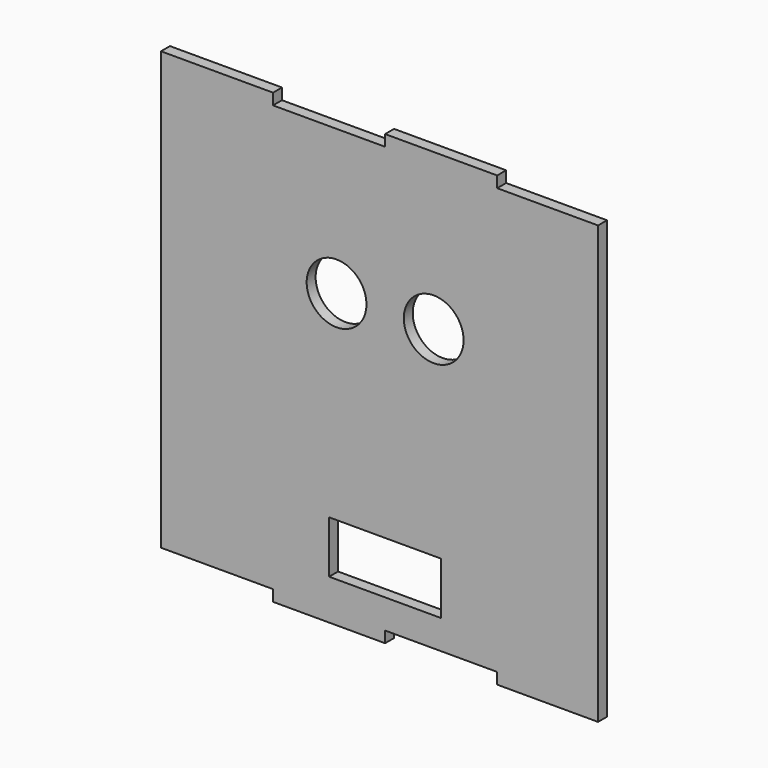
from build123d import *

# Parameters (mm, degrees)
F0_W     = 30
F0_H     = 14
F0_R     = 8
F1_DEPTH = 1.5


# Not quite as in the source:
# - a feature names something its author has since deleted; it is built from what else it names


with BuildPart() as f1:
    # F0 (on Front) → F1 (new body, symmetric)
    with BuildSketch(Plane.XZ):
        Polygon((-30, -2.9994321861), (0, -2.9994321861), (0, 0), (30, 0), (30, -2.9994321861), (57, -2.9994321861), (57, 114.0005678139), (30, 114.0005678139), (30, 117.0005678139), (0, 117.0005678139), (0, 114.0005678139), (-30, 114.0005678139), (-30, 117.0005678139), (-60, 117.0005678139), (-60, 0), (-30, 0), align=None)
        with Locations((0, 14.8116284981)):
            Rectangle(F0_W, F0_H, mode=Mode.SUBTRACT)
        with Locations((-13, 75.2281695604)):
            Circle(F0_R, mode=Mode.SUBTRACT)
        with Locations((13, 75.2218647463)):
            Circle(F0_R, mode=Mode.SUBTRACT)
    extrude(amount=F1_DEPTH, both=True)


solid = f1.part
